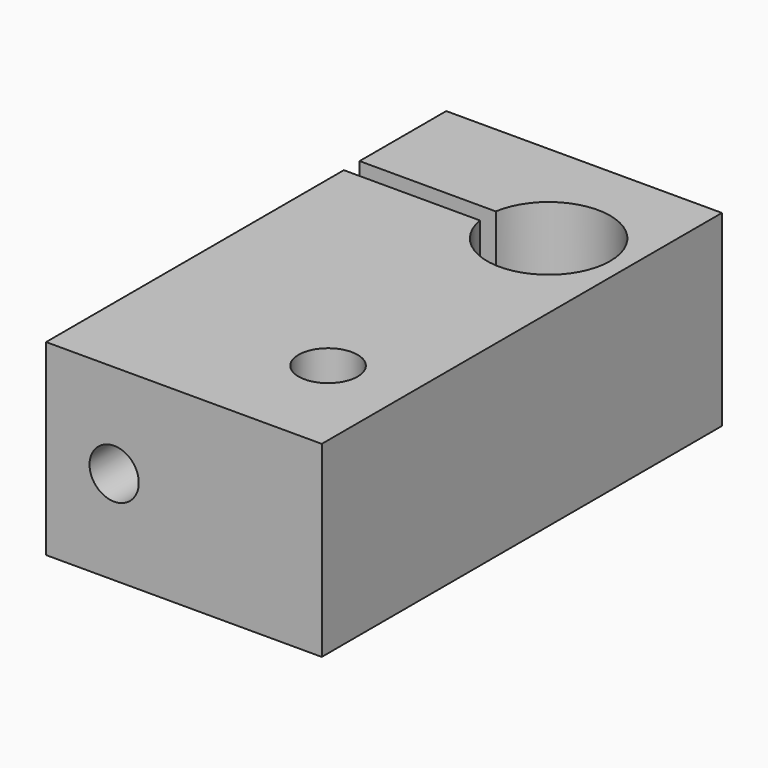
from build123d import *

# Parameters (mm, degrees)
F0_R     = 1.5
F1_DEPTH = 9.525
F2_R     = 1.25
F3_DEPTH = 25.401


# Not quite as in the source:
# - a length typed as a fraction of an inch, garbled in the dataset ("3 / 203.2 mm" for 3/8 in), is restored


with BuildPart() as f1:
    # F0 (on Top) → F1 (new body)
    with BuildSketch(Plane.XY):
        with BuildLine():
            Line((-7, -12.7), (7, -12.7))
            Line((7, -12.7), (7, 12.7))
            Line((7, 12.7), (-7, 12.7))
            Line((-7, 12.7), (-7, 7.2))
            Line((-7, 7.2), (-0.0847406698, 7.2))
            ThreePointArc((-0.0847406698, 7.2), (6.125, 6.7), (-0.0847406698, 6.2))
            Line((-0.0847406698, 6.2), (-7, 6.2))
            Line((-7, 6.2), (-7, -12.7))
        make_face()
        with Locations((3, -7.3)):
            Circle(F0_R, mode=Mode.SUBTRACT)
    extrude(amount=F1_DEPTH)

    # F2 (on face) → F3 (cut, through all)
    with BuildSketch(Plane(origin=(0, 12.7, 0), x_dir=(-1, 0, 0), z_dir=(0, 1, 0))):
        with Locations((3.5423703349, 4.7625)):
            Circle(F2_R)
    extrude(amount=-F3_DEPTH, mode=Mode.SUBTRACT)


solid = f1.part
